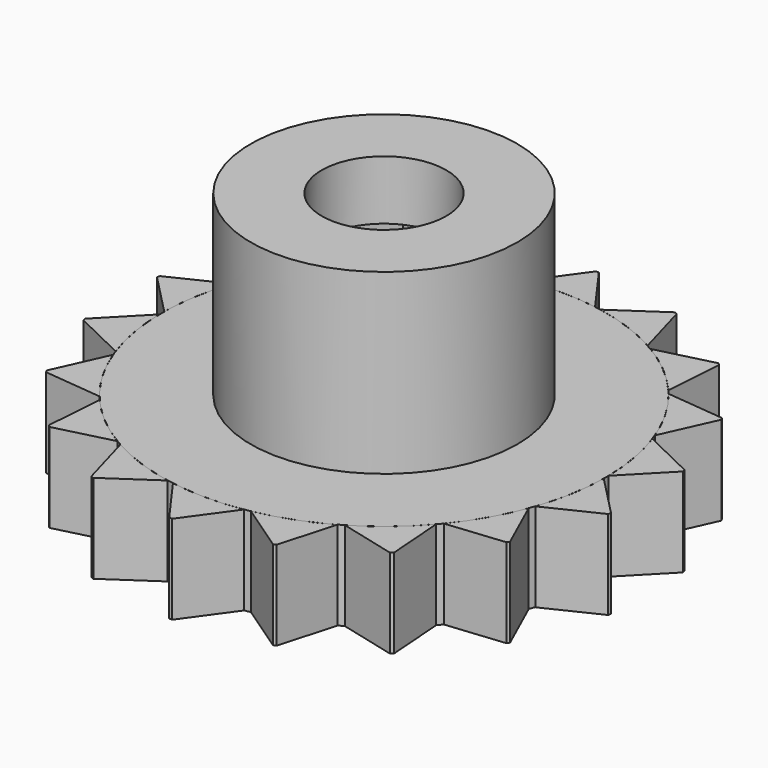
from build123d import *

# Parameters (mm, degrees)
F0_R     = 4.5
F0_R_2   = 2.1
F1_DEPTH = 9
F0_R_3   = 7.5
F2_DEPTH = 3
F3_START = 4.6
F3_DEPTH = 2.4
F5_DEPTH = 3
F6_COUNT = 18


# Not quite as in the source:
# - a feature names something its author has since deleted; it is built from what else it names


with BuildPart() as f1:
    # F0 (on Top) → F1 (new body)
    with BuildSketch(Plane.XY):
        Circle(F0_R)
        Polygon((3.2908965344, 0), (1.6454482672, -2.85), (-1.6454482672, -2.85), (-3.2908965344, 0), (-1.6454482672, 2.85), (1.6454482672, 2.85), align=None, mode=Mode.SUBTRACT)
        Polygon((-1.6454482672, -2.85), (1.6454482672, -2.85), (3.2908965344, 0), (1.6454482672, 2.85), (-1.6454482672, 2.85), (-3.2908965344, 0), align=None)
        Circle(F0_R_2, mode=Mode.SUBTRACT)
    extrude(amount=F1_DEPTH)

    # F0 (on Top) → F2 (join)
    with BuildSketch(Plane.XY):
        Circle(F0_R_3)
        Circle(F0_R, mode=Mode.SUBTRACT)
    extrude(amount=F2_DEPTH)

    # F0 (on Top) → F3 (cut)
    with BuildSketch(Plane.XY.offset(F3_START)):
        Polygon((-1.6454482672, -2.85), (1.6454482672, -2.85), (3.2908965344, 0), (1.6454482672, 2.85), (-1.6454482672, 2.85), (-3.2908965344, 0), align=None)
        Circle(F0_R_2, mode=Mode.SUBTRACT)
    extrude(amount=F3_DEPTH, mode=Mode.SUBTRACT)


with BuildPart() as f5:
    # F4 (on face) → F5 (new body, through all)
    with BuildSketch(Plane.XY.offset(3)):
        with BuildLine():
            ThreePointArc((1.2, -7.4033776076), (0, -7.5), (-1.2, -7.4033776076))
            Line((-1.2, -7.4033776076), (-0.05, -9))
            Line((-0.05, -9), (0.05, -9))
            Line((0.05, -9), (1.2, -7.4033776076))
        make_face()
    extrude(amount=-F5_DEPTH)


with BuildPart() as f6_1:
    # F6: instance of F5
    add(f5.part.rotate(Axis((0, 0, 0), (0, 0, -1)), 1 * 360 / F6_COUNT))


with BuildPart() as f6_2:
    # F6: instance of F5
    add(f5.part.rotate(Axis((0, 0, 0), (0, 0, -1)), 2 * 360 / F6_COUNT))


with BuildPart() as f6_3:
    # F6: instance of F5
    add(f5.part.rotate(Axis((0, 0, 0), (0, 0, -1)), 3 * 360 / F6_COUNT))


with BuildPart() as f6_4:
    # F6: instance of F5
    add(f5.part.rotate(Axis((0, 0, 0), (0, 0, -1)), 4 * 360 / F6_COUNT))


with BuildPart() as f6_5:
    # F6: instance of F5
    add(f5.part.rotate(Axis((0, 0, 0), (0, 0, -1)), 5 * 360 / F6_COUNT))


with BuildPart() as f6_6:
    # F6: instance of F5
    add(f5.part.rotate(Axis((0, 0, 0), (0, 0, -1)), 6 * 360 / F6_COUNT))


with BuildPart() as f6_7:
    # F6: instance of F5
    add(f5.part.rotate(Axis((0, 0, 0), (0, 0, -1)), 7 * 360 / F6_COUNT))


with BuildPart() as f6_8:
    # F6: instance of F5
    add(f5.part.rotate(Axis((0, 0, 0), (0, 0, -1)), 8 * 360 / F6_COUNT))


with BuildPart() as f6_9:
    # F6: instance of F5
    add(f5.part.rotate(Axis((0, 0, 0), (0, 0, -1)), 9 * 360 / F6_COUNT))


with BuildPart() as f6_10:
    # F6: instance of F5
    add(f5.part.rotate(Axis((0, 0, 0), (0, 0, -1)), 10 * 360 / F6_COUNT))


with BuildPart() as f6_11:
    # F6: instance of F5
    add(f5.part.rotate(Axis((0, 0, 0), (0, 0, -1)), 11 * 360 / F6_COUNT))


with BuildPart() as f6_12:
    # F6: instance of F5
    add(f5.part.rotate(Axis((0, 0, 0), (0, 0, -1)), 12 * 360 / F6_COUNT))


with BuildPart() as f6_13:
    # F6: instance of F5
    add(f5.part.rotate(Axis((0, 0, 0), (0, 0, -1)), 13 * 360 / F6_COUNT))


with BuildPart() as f6_14:
    # F6: instance of F5
    add(f5.part.rotate(Axis((0, 0, 0), (0, 0, -1)), 14 * 360 / F6_COUNT))


with BuildPart() as f6_15:
    # F6: instance of F5
    add(f5.part.rotate(Axis((0, 0, 0), (0, 0, -1)), 15 * 360 / F6_COUNT))


with BuildPart() as f6_16:
    # F6: instance of F5
    add(f5.part.rotate(Axis((0, 0, 0), (0, 0, -1)), 16 * 360 / F6_COUNT))


with BuildPart() as f6_17:
    # F6: instance of F5
    add(f5.part.rotate(Axis((0, 0, 0), (0, 0, -1)), 17 * 360 / F6_COUNT))


solid = Compound([f1.part, f5.part, f6_1.part, f6_2.part, f6_3.part, f6_4.part, f6_5.part, f6_6.part, f6_7.part, f6_8.part, f6_9.part, f6_10.part, f6_11.part, f6_12.part, f6_13.part, f6_14.part, f6_15.part, f6_16.part, f6_17.part])
